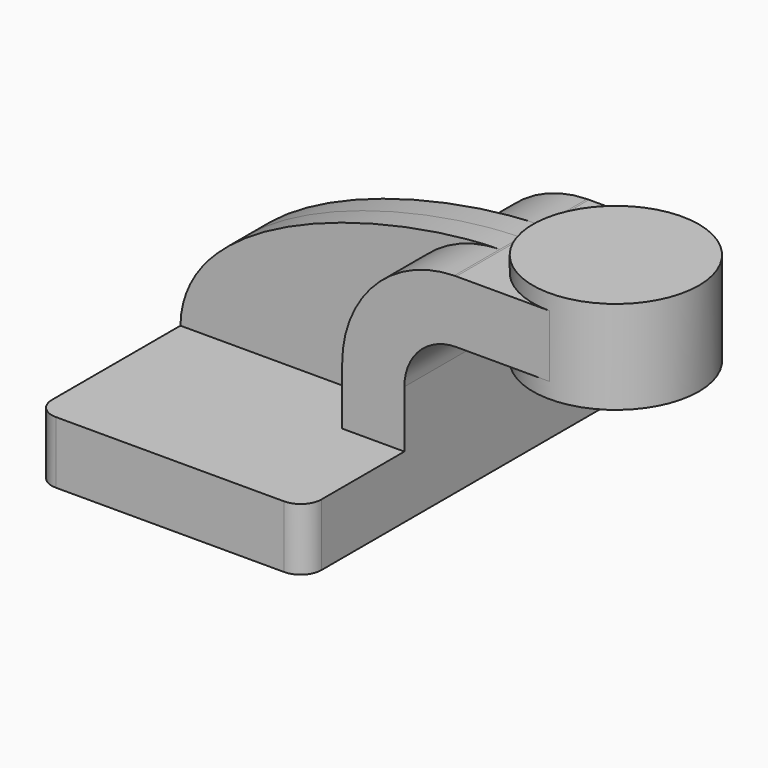
from build123d import *

# Parameters (mm, degrees)
F1_DEPTH = 63.5
F0_W     = 25.4
F0_H     = 19.05
F2_DEPTH = 25.4
F3_DEPTH = 7.9375
F5_R     = 6.35


with BuildPart() as f1:
    # F0 (on Front) → F1 (new body, symmetric)
    with BuildSketch(Plane.XZ):
        Polygon((41.275, -9.525), (41.275, 9.525), (22.225, 9.525), (-41.275, 9.525), (-41.275, -9.525), align=None)
    extrude(amount=F1_DEPTH, both=True)

    # F0 (on Front) → F2 (join, symmetric)
    with BuildSketch(Plane.XZ):
        with BuildLine():
            Line((22.225, 9.525), (41.275, 9.525))
            Line((41.275, 9.525), (41.275, 27.0002))
            ThreePointArc((41.275, 27.0002), (45.9246798487, 38.2255201513), (57.15, 42.8752))
            Line((57.15, 42.8752), (60.325, 42.8752))
            Line((60.325, 42.8752), (60.325, 61.9252))
            Line((60.325, 61.9252), (57.15, 61.9252))
            add(Edge.make_bspline(
                [(56.5697529207, 61.9203795288), (56.7642060535, 61.9225634714), (56.9576279056, 61.9241702866), (57.15, 61.9252)],
                knots=[110.8594899862, 110.8594899862, 110.8594899862, 110.8594899862, 111.5045361635, 111.5045361635, 111.5045361635, 111.5045361635], degree=3))
            ThreePointArc((56.5697529207, 61.9203795288), (32.2499924273, 51.4898967698), (22.225, 27.0002))
            Line((22.225, 27.0002), (22.225, 9.525))
        make_face()
        Polygon((41.275, -9.525), (41.275, 9.525), (22.225, 9.525), (-41.275, 9.525), (-41.275, -9.525), align=None)
        with Locations((73.025, 52.4002)):
            Rectangle(F0_W, F0_H)
    extrude(amount=F2_DEPTH, both=True)

    # F0 (on Front) → F3 (join, symmetric)
    with BuildSketch(Plane.XZ):
        with BuildLine():
            Line((-41.275, 9.525), (22.225, 9.525))
            Line((22.225, 9.525), (22.225, 27.0002))
            ThreePointArc((22.225, 27.0002), (32.2499924273, 51.4898967698), (56.5697529207, 61.9203795288))
            add(Edge.make_bspline(
                [(-41.275, 9.525), (-40.7295745203, 44.1231784774), (23.1504786353, 61.5450408791), (56.5697529207, 61.9203795288)],
                knots=[0, 0, 0, 0, 110.8594899862, 110.8594899862, 110.8594899862, 110.8594899862], degree=3))
        make_face()
    extrude(amount=F3_DEPTH, both=True)

    # F0 (on Front) → F4 (revolve)
    with BuildSketch(Plane.XZ):
        Polygon((85.725, 61.9252), (85.725, 42.8752), (85.725, 38.1), (111.125, 38.1), (111.125, 66.675), (85.725, 66.675), align=None)
    revolve(axis=Axis((85.725, 0, 52.3875), (0, 0, 1)))

    # F5
    f5_edges = [f1.edges().sort_by_distance(p)[0] for p in [
        (-41.275, -63.5, 0),
        (41.275, -63.5, 0),
        (41.275, 63.5, 0),
        (-41.275, 63.5, 0),
    ]]
    fillet(f5_edges, radius=F5_R)


solid = f1.part
